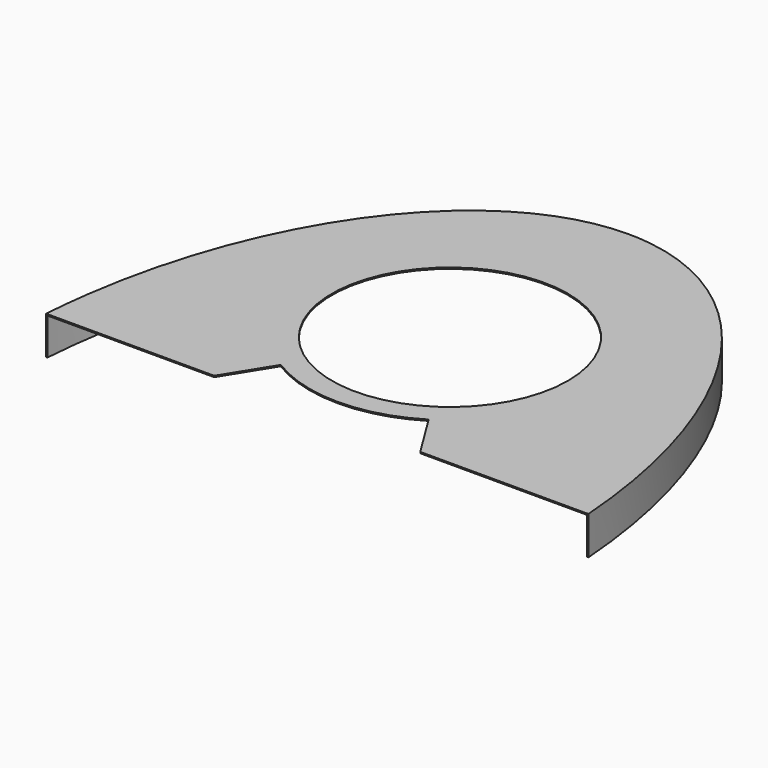
from build123d import *

# Parameters (mm, degrees)
F0_R     = 925
F1_DEPTH = 300
F2_T     = -10


with BuildPart() as f1:
    # F0 (on Top) → F1 (new body)
    with BuildSketch(Plane.XY):
        with BuildLine():
            add(Edge.make_bspline(
                [(0, 1525.044003), (-1902.67853, 1525.044003), (-2125, -1524.955997)],
                knots=[0, 0, 0, 1.453682, 1.453682, 1.453682], degree=2, weights=[1, 0.747277, 1]))
            Line((-2125, -1524.955997), (-807.5, -1524.955997))
            Line((-807.5, -1524.955997), (-579.5, -1157.897173))
            ThreePointArc((-579.5, -1157.897173), (0, -1323.227133), (579.5, -1157.897173))
            Line((579.5, -1157.897173), (807.5, -1524.955997))
            Line((807.5, -1524.955997), (2125, -1524.955997))
            add(Edge.make_bspline(
                [(2125, -1524.955997), (1902.67853, 1525.044004), (0, 1525.044003)],
                knots=[4.829503, 4.829503, 4.829503, 6.283185, 6.283185, 6.283185], degree=2, weights=[1, 0.747277, 1]))
        make_face()
        with Locations((0, -224.955997)):
            Circle(F0_R, mode=Mode.SUBTRACT)
    extrude(amount=F1_DEPTH)

    # F2
    f2_openings = [f1.faces().sort_by_distance(p)[0] for p in [
        (0, -1270.915566, 0),
        (0, -1323.227133, 150),
        (-693.5, -1341.426585, 150),
        (-1466.25, -1524.955997, 150),
        (1466.25, -1524.955997, 150),
        (693.5, -1341.426585, 150),
        (-925, -224.955997, 150),
    ]]
    offset(amount=F2_T, openings=f2_openings)


solid = f1.part
